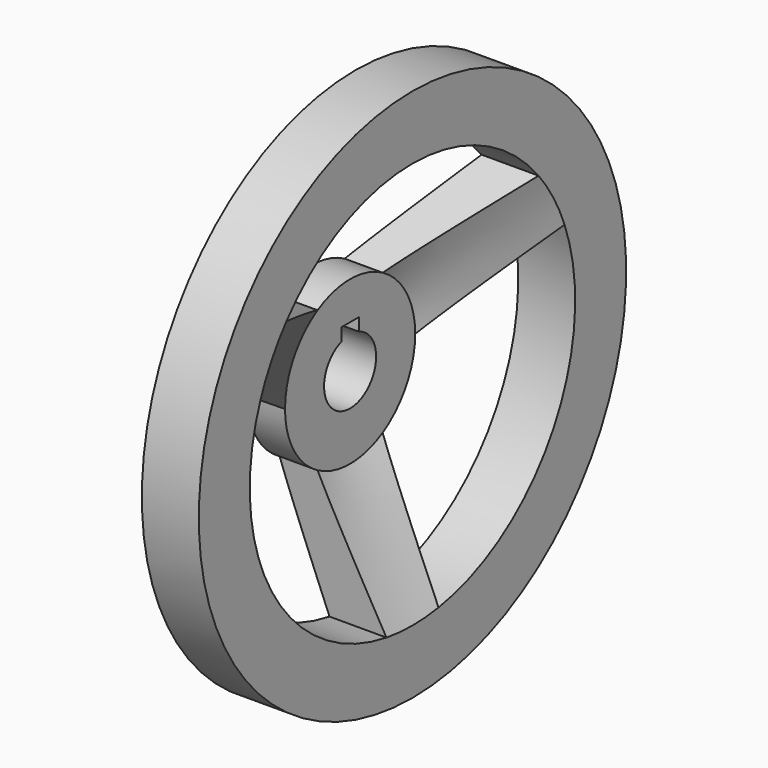
from build123d import *

# Parameters (mm, degrees)
F2_W            = 4
F2_H            = 8
F3_DEPTH        = 25
F5_DEPTH        = 28.501
F5_COPIES_COUNT = 3


# Not quite as in the source:
# - a pattern or mirror of a feature is missing from the dataset's text; its kind, count and spacing are read off the source's solid


with BuildPart() as f1:
    # F0 (on Front) → F1 (revolve)
    with BuildSketch(Plane.XZ):
        Polygon((0, 11), (0, 6), (17, 6), (17, 15), (28.5, 37.5), (28.5, 49.25), (18, 49.25), (18, 37.5), (10, 15), (10, 11), align=None)
    revolve(axis=Axis((-9.663007474, 0, 0), (-1, 0, 0)))

    # F2 (on Right) → F3 (cut)
    with BuildSketch(Plane.YZ):
        with Locations((0, 4)):
            Rectangle(F2_W, F2_H)
    extrude(amount=F3_DEPTH, mode=Mode.SUBTRACT)

    # F4 (on face) → F5 (cut, through all)
    with BuildSketch(Plane.YZ.offset(28.5)):
        with BuildLine():
            Line((7.5, 12.9903810568), (29.0575654097, 23.7045964416))
            ThreePointArc((29.0575654097, 23.7045964416), (0, 37.5), (-29.0575654097, 23.7045964416))
            Line((-29.0575654097, 23.7045964416), (-7.5, 12.9903810568))
            ThreePointArc((-7.5, 12.9903810568), (0, 15), (7.5, 12.9903810568))
        make_face()
    f5 = extrude(amount=-F5_DEPTH, mode=Mode.SUBTRACT)

    # F5_copies: F5 ×3 about axis
    f5_copies_axis = Axis((0, 0, 0), (1, 0, 0))
    for i in range(1, F5_COPIES_COUNT):
        add(f5.rotate(f5_copies_axis, i * 360 / F5_COPIES_COUNT), mode=Mode.SUBTRACT)


solid = f1.part
